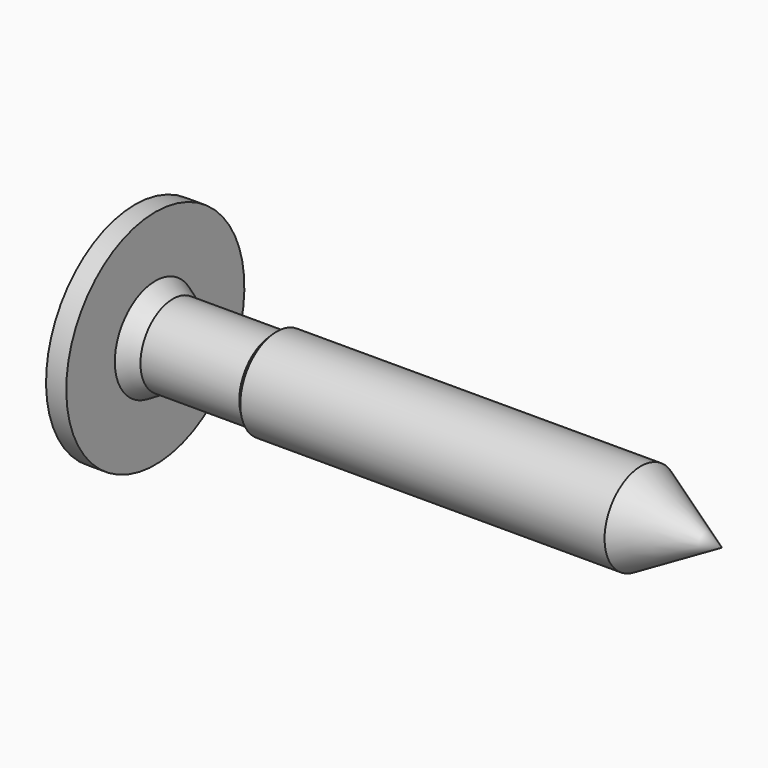
from build123d import *

# Parameters (mm, degrees)
F3_DEPTH = 0.5


# Not quite as in the source:
# - a pattern or mirror of a feature is missing from the dataset's text; its kind, count and spacing are read off the source's solid


with BuildPart() as f1:
    # F0 (on Front) → F1 (revolve)
    with BuildSketch(Plane.XZ):
        with BuildLine():
            Line((28, 0), (24, 2.25))
            Line((24, 2.25), (6, 2.25))
            Line((6, 2.25), (5.75, 2))
            Line((5.75, 2), (0.8660254038, 2))
            Line((0.8660254038, 2), (0, 2.5))
            Line((0, 2.5), (0, 5.5))
            Line((0, 5.5), (-1, 5.5))
            Line((-1, 5.5), (-1, 4.5))
            ThreePointArc((-1, 4.5), (-1.7469875145, 2.3048861143), (-2, 0))
            Line((-2, 0), (28, 0))
        make_face()
    revolve(axis=Axis((13, 0, 0), (-1, 0, 0)))

    # F2 (on Front) → F3 (cut, symmetric)
    with BuildSketch(Plane.XZ):
        Polygon((-1.7016947762, 2.5), (-2, 2.5), (-2, 0), (-2, -2.5), (-1.7016947762, -2.5), (0.5, -0.5), (0.5, 0), (0.5, 0.5), align=None)
    f3 = extrude(amount=F3_DEPTH, both=True, mode=Mode.SUBTRACT)

    # F3_copies: F3 across plane
    add(f3.mirror(Plane(origin=(0, 0, 0), x_dir=(0, -0.7071067802, -0.7071067821), z_dir=(-2.1e-09, -0.7071067821, 0.7071067802))), mode=Mode.SUBTRACT)


solid = f1.part
